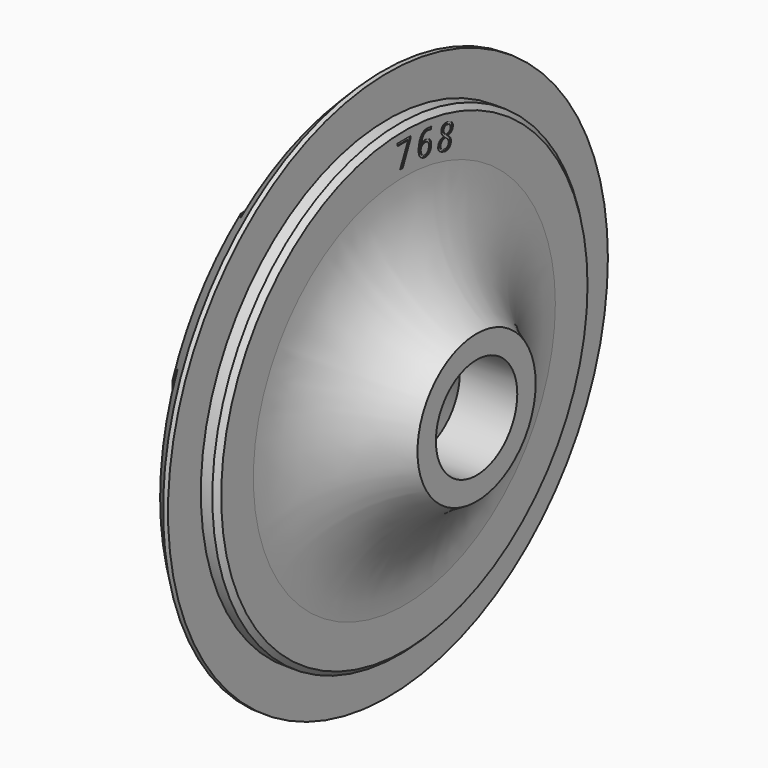
from build123d import *

# Parameters (mm, degrees)
F2_SIZE      = 1.3
F4_DEPTH     = 0.4
F5_T1_DEPTH  = 0.4
F5_T3_DEPTH  = 1.1640297733
F6_TEXT_SIZE = 2.0833333333
F7_DEPTH     = 0.05
F8_SIZE      = 0.3
F9_SIZE      = 0.1


# Not quite as in the source:
# - a fillet or chamfer that OpenCascade refuses, or shapes differently, is made with other operations: its cross-section is extruded or revolved along the edge and cut away or added
# - Text() gives the source's letters only with a copy of the font that has no kerning and outlines rounded to 1/6400 em; it was checked with that copy


with BuildPart() as f1:
    # F0 (on Top) → F1 (revolve)
    with BuildSketch(Plane.XY):
        with BuildLine():
            Line((-4.4, 11.5), (-4.4, 14.25))
            Line((-4.4, 14.25), (-5.4, 14.25))
            Line((-5.4, 14.25), (-5.4, 16.75))
            Line((-5.4, 16.75), (-7, 16.75))
            Line((-7, 16.75), (-7, 6))
            Line((-7, 6), (-6.4, 6))
            Line((-6.4, 6), (-3.5, 3.1))
            Line((-3.5, 3.1), (0, 3.1))
            Line((0, 3.1), (0, 4.5))
            ThreePointArc((0, 4.5), (-3.20864483, 7.3659946783), (-4.4, 11.5))
        make_face()
    revolve(axis=Axis((-3.5, 0, 0), (-1, 0, 0)))

    # F2
    f2_edges = [f1.edges().sort_by_distance(p)[0] for p in [
        (-7, -16.75, 0),
    ]]
    chamfer(f2_edges, length=F2_SIZE)

    # F3 (on face) → F4 (cut)
    with BuildSketch(Plane(origin=(-7, 0, 0), x_dir=(0, -1, 0), z_dir=(-1, 0, 0))):
        with BuildLine():
            ThreePointArc((14.5, -8.3852549156), (16.1777238819, -4.3409388385), (16.75, 0))
            ThreePointArc((16.75, 0), (16.1777238819, 4.3409388385), (14.5, 8.3852549156))
            Line((14.5, 8.3852549156), (14.5, 5.3340884882))
            ThreePointArc((14.5, 5.3340884882), (15.2106459429, 2.7090127353), (15.45, 0))
            ThreePointArc((15.45, 0), (15.2106459429, -2.7090127353), (14.5, -5.3340884882))
            Line((14.5, -5.3340884882), (14.5, -8.3852549156))
        make_face()
        with BuildLine():
            Line((9.0803358969, 12.5), (11.1495515605, 12.5))
            ThreePointArc((11.1495515605, 12.5), (0, 16.75), (-11.1495515605, 12.5))
            Line((-11.1495515605, 12.5), (-9.0803358969, 12.5))
            ThreePointArc((-9.0803358969, 12.5), (0, 15.45), (9.0803358969, 12.5))
        make_face()
        with BuildLine():
            ThreePointArc((15.45, 0), (15.2106459429, 2.7090127353), (14.5, 5.3340884882))
            Line((14.5, 5.3340884882), (14.5, -5.3340884882))
            ThreePointArc((14.5, -5.3340884882), (15.2106459429, -2.7090127353), (15.45, 0))
        make_face()
        with BuildLine():
            ThreePointArc((2.9, -16.49704519), (5.9018735713, -15.6757898796), (8.7, -14.3133678776))
            Line((8.7, -14.3133678776), (8.7, -12.7676348632))
            ThreePointArc((8.7, -12.7676348632), (5.9236241205, -14.2693089279), (2.9, -15.1753912635))
            Line((2.9, -15.1753912635), (2.9, -16.49704519))
        make_face()
        with BuildLine():
            Line((8.7, 12.5), (9.0803358969, 12.5))
            ThreePointArc((9.0803358969, 12.5), (0, 15.45), (-9.0803358969, 12.5))
            Line((-9.0803358969, 12.5), (-8.7, 12.5))
            Line((-8.7, 12.5), (-4.9428840308, 6.2471089796))
            ThreePointArc((-4.9428840308, 6.2471089796), (-3.7060377863, 5.7536573635), (-2.9, 6.813650862))
            Line((-2.9, 6.813650862), (-2.9, 12.5))
            Line((-2.9, 12.5), (2.9, 12.5))
            Line((2.9, 12.5), (2.9, 6.813650862))
            ThreePointArc((2.9, 6.813650862), (3.7060377863, 5.7536573635), (4.9428840308, 6.2471089796))
            Line((4.9428840308, 6.2471089796), (8.7, 12.5))
        make_face()
        with BuildLine():
            ThreePointArc((2.9, -15.1753912635), (5.9236241205, -14.2693089279), (8.7, -12.7676348632))
            Line((8.7, -12.7676348632), (8.7, 1.2386966468))
            Line((8.7, 1.2386966468), (2.9, -8.4141243508))
            Line((2.9, -8.4141243508), (2.9, -15.1753912635))
        make_face()
        with BuildLine():
            Line((-14.5, 5.3340884882), (-14.5, 8.3852549156))
            ThreePointArc((-14.5, 8.3852549156), (-16.75, 0), (-14.5, -8.3852549156))
            Line((-14.5, -8.3852549156), (-14.5, -5.3340884882))
            ThreePointArc((-14.5, -5.3340884882), (-15.45, 0), (-14.5, 5.3340884882))
        make_face()
        with BuildLine():
            ThreePointArc((-8.7, -14.3133678776), (-5.9018735713, -15.6757898796), (-2.9, -16.49704519))
            Line((-2.9, -16.49704519), (-2.9, -15.1753912635))
            ThreePointArc((-2.9, -15.1753912635), (-5.9236241205, -14.2693089279), (-8.7, -12.7676348632))
            Line((-8.7, -12.7676348632), (-8.7, -14.3133678776))
        make_face()
        with BuildLine():
            Line((-14.5, -5.3340884882), (-14.5, 5.3340884882))
            ThreePointArc((-14.5, 5.3340884882), (-15.45, 0), (-14.5, -5.3340884882))
        make_face()
        with BuildLine():
            ThreePointArc((-8.7, -12.7676348632), (-5.9236241205, -14.2693089279), (-2.9, -15.1753912635))
            Line((-2.9, -15.1753912635), (-2.9, -8.4141243508))
            Line((-2.9, -8.4141243508), (-8.7, 1.2386966468))
            Line((-8.7, 1.2386966468), (-8.7, -12.7676348632))
        make_face()
    extrude(amount=-F4_DEPTH, mode=Mode.SUBTRACT)

    # F5: fillet of radius 1.1 on 4 edges, made by hand

    # F5_s2 → F5_t1 (join)
    with BuildSketch(Plane.YZ.offset(-7)):
        with BuildLine():
            ThreePointArc((8.7004, -2.7283019394), (7.8939620715, -1.6677822271), (6.6565018181, -2.161478808))
            Line((6.6565018181, -2.161478808), (6.5621666073, -2.1047964949))
            ThreePointArc((6.5621666073, -2.1047964949), (7.5840871317, -0.4048117751), (8.6056647892, 1.29537896))
            Line((8.6056647892, 1.29537896), (8.8100546074, 1.2386966468))
            ThreePointArc((8.8100546074, 1.2386966468), (8.8100546074, -0.7448026463), (8.8104546074, -2.7283019394))
            Line((8.8104546074, -2.7283019394), (8.7004, -2.7283019394))
        make_face()
        with BuildLine():
            ThreePointArc((-8.7004, -2.7283019394), (-7.8939620715, -1.6677822271), (-6.6565018181, -2.161478808))
            Line((-6.6565018181, -2.161478808), (-6.5621666073, -2.1047964949))
            ThreePointArc((-6.5621666073, -2.1047964949), (-7.5840871317, -0.4048117751), (-8.6056647892, 1.29537896))
            Line((-8.6056647892, 1.29537896), (-8.8100546074, 1.2386966468))
            ThreePointArc((-8.8100546074, 1.2386966468), (-8.8100546074, -0.7448026463), (-8.8104546074, -2.7283019394))
            Line((-8.8104546074, -2.7283019394), (-8.7004, -2.7283019394))
        make_face()
    extrude(amount=F5_T1_DEPTH)

    # F5_s4 → F5_t3 (join)
    with BuildSketch(Plane.YZ.offset(-7)):
        with BuildLine():
            ThreePointArc((2.8996, -8.7197359984), (2.9396937884, -8.4251324126), (3.0570587677, -8.1519580246))
            Line((3.0570587677, -8.1519580246), (2.9625646445, -8.0951802272))
            ThreePointArc((2.9625646445, -8.0951802272), (2.8842066941, -8.2263663979), (2.8055058768, -8.3573465534))
            Line((2.8055058768, -8.3573465534), (2.78976, -8.4141243508))
            ThreePointArc((2.78976, -8.4141243508), (2.78976, -8.5669301746), (2.78936, -8.7197359984))
            Line((2.78936, -8.7197359984), (2.8996, -8.7197359984))
        make_face()
        with BuildLine():
            ThreePointArc((-2.8996, -8.7197359984), (-2.9396937884, -8.4251324126), (-3.0570587677, -8.1519580246))
            Line((-3.0570587677, -8.1519580246), (-2.9625646445, -8.0951802272))
            ThreePointArc((-2.9625646445, -8.0951802272), (-2.8842066941, -8.2263663979), (-2.8055058768, -8.3573465534))
            Line((-2.8055058768, -8.3573465534), (-2.78976, -8.4141243508))
            ThreePointArc((-2.78976, -8.4141243508), (-2.78976, -8.5669301746), (-2.78936, -8.7197359984))
            Line((-2.78936, -8.7197359984), (-2.8996, -8.7197359984))
        make_face()
    extrude(amount=F5_T3_DEPTH)

    # F6 (on face) → F7 (cut)
    with BuildSketch(Plane.YZ.offset(-4.4)):
        with Locations((-0.6101888021, 12)):
            Text('7', F6_TEXT_SIZE, font='Open Sans', text_align=(TextAlign.LEFT, TextAlign.BOTTOM))
        with BuildLine():
            add(Edge.make_bspline(
                [(1.3911920227, 11.9124736168), (1.2492672408, 11.965505738), (1.168086207, 12.102022835)],
                knots=[0.2780169607, 0.2780169607, 0.2780169607, 1, 1, 1], degree=2))
            Line((1.3911920227, 11.9124736168), (1.5039988028, 11.9053764158))
            Line((1.5039988028, 11.9053764158), (1.6329910314, 11.8807698321))
            add(Edge.make_bspline(
                [(1.8658957751, 11.9728554781), (1.7668517571, 11.8921760098), (1.6329910314, 11.8807698321)],
                knots=[0, 0, 0, 0.6961452699, 0.6961452699, 0.6961452699], degree=2))
            add(Edge.make_bspline(
                [(2.0372600894, 12.3190162698), (2.0081707028, 12.0887500648), (1.8658957751, 11.9728554781)],
                knots=[0, 0, 0, 1, 1, 1], degree=2))
            add(Edge.make_bspline(
                [(1.9639386607, 12.6593399563), (2.063248784, 12.5247379706), (2.0372600894, 12.3190162698)],
                knots=[0, 0, 0, 1, 1, 1], degree=2))
            add(Edge.make_bspline(
                [(1.6656888708, 12.8190738665), (1.8646285374, 12.7939419421), (1.9639386607, 12.6593399563)],
                knots=[0, 0, 0, 1, 1, 1], degree=2))
            add(Edge.make_bspline(
                [(1.2923652787, 12.6897134657), (1.4254110915, 12.849428009), (1.6656888708, 12.8190738665)],
                knots=[0, 0, 0, 1, 1, 1], degree=2))
            Line((1.2923652787, 12.6897134657), (1.2804159806, 12.6912230132))
            add(Edge.make_bspline(
                [(1.4762395094, 13.1387963058), (1.332429483, 13.006854298), (1.2804159806, 12.6912230132)],
                knots=[0, 0, 0, 1, 1, 1], degree=2))
            add(Edge.make_bspline(
                [(1.8574207289, 13.2407513582), (1.6200495358, 13.2707383135), (1.4762395094, 13.1387963058)],
                knots=[0, 0, 0, 1, 1, 1], degree=2))
            add(Edge.make_bspline(
                [(2.0318631422, 13.1931217276), (1.9572135163, 13.2281445974), (1.8574207289, 13.2407513582)],
                knots=[0, 0, 0, 1, 1, 1], degree=2))
            Line((2.0318631422, 13.1931217276), (2.0501001068, 13.3374821676))
            add(Edge.make_bspline(
                [(1.8729447966, 13.3792204636), (1.9869475601, 13.3648185653), (2.0501001068, 13.3374821676)],
                knots=[0, 0, 0, 1, 1, 1], degree=2))
            add(Edge.make_bspline(
                [(1.3456378689, 13.2269867417), (1.5419169421, 13.4210390067), (1.8729447966, 13.3792204636)],
                knots=[0, 0, 0, 1, 1, 1], degree=2))
            add(Edge.make_bspline(
                [(1.0944031103, 12.5979154329), (1.1493587957, 13.0329344767), (1.3456378689, 13.2269867417)],
                knots=[0, 0, 0, 1, 1, 1], degree=2))
            add(Edge.make_bspline(
                [(1.168086207, 12.102022835), (1.0556444606, 12.2911091288), (1.0944031103, 12.5979154329)],
                knots=[0, 0, 0, 1, 1, 1], degree=2))
        make_face()
        with BuildLine():
            add(Edge.make_bspline(
                [(1.5255567916, 12.0266778564), (1.6689483695, 12.0085632875), (1.7594957026, 12.088994757)],
                knots=[0, 0, 0, 1, 1, 1], degree=2))
            add(Edge.make_bspline(
                [(1.3631201393, 12.100515938), (1.4306083143, 12.0386726385), (1.5255567916, 12.0266778564)],
                knots=[0, 0, 0, 1, 1, 1], degree=2))
            add(Edge.make_bspline(
                [(1.2666047187, 12.2572402731), (1.2956319644, 12.1623592375), (1.3631201393, 12.100515938)],
                knots=[0, 0, 0, 1, 1, 1], degree=2))
            add(Edge.make_bspline(
                [(1.2507146153, 12.456112498), (1.237577473, 12.3521213086), (1.2666047187, 12.2572402731)],
                knots=[0, 0, 0, 1, 1, 1], degree=2))
            add(Edge.make_bspline(
                [(1.3128222221, 12.5867280854), (1.259649504, 12.526839425), (1.2507146153, 12.456112498)],
                knots=[0, 0, 0, 1, 1, 1], degree=2))
            add(Edge.make_bspline(
                [(1.4464602893, 12.6745121437), (1.3659949402, 12.6466167459), (1.3128222221, 12.5867280854)],
                knots=[0, 0, 0, 1, 1, 1], degree=2))
            add(Edge.make_bspline(
                [(1.6176757137, 12.6909431409), (1.5269256385, 12.7024075415), (1.4464602893, 12.6745121437)],
                knots=[0, 0, 0, 1, 1, 1], degree=2))
            add(Edge.make_bspline(
                [(1.8270201595, 12.5793527447), (1.7639738776, 12.6724613848), (1.6176757137, 12.6909431409)],
                knots=[0, 0, 0, 1, 1, 1], degree=2))
            add(Edge.make_bspline(
                [(1.8715846852, 12.3399459407), (1.8900664413, 12.4862441047), (1.8270201595, 12.5793527447)],
                knots=[0, 0, 0, 1, 1, 1], degree=2))
            add(Edge.make_bspline(
                [(1.7594957026, 12.088994757), (1.8500430357, 12.1694262264), (1.8715846852, 12.3399459407)],
                knots=[0, 0, 0, 1, 1, 1], degree=2))
        make_face(mode=Mode.SUBTRACT)
        with BuildLine():
            Line((2.984278646, 11.6229979335), (3.1084826292, 11.582641613))
            add(Edge.make_bspline(
                [(3.3407163455, 11.6244062371), (3.239004536, 11.5744991717), (3.1084826292, 11.582641613)],
                knots=[0, 0, 0, 0.666283244, 0.666283244, 0.666283244], degree=2))
            add(Edge.make_bspline(
                [(3.5393535811, 11.8783969056), (3.4933718571, 11.6993099149), (3.3407163455, 11.6244062371)],
                knots=[0, 0, 0, 1, 1, 1], degree=2))
            add(Edge.make_bspline(
                [(3.5202228201, 12.1108345939), (3.5705207707, 11.9997850947), (3.5393535811, 11.8783969056)],
                knots=[0, 0, 0, 1, 1, 1], degree=2))
            add(Edge.make_bspline(
                [(3.3161551014, 12.3507625756), (3.4699248695, 12.2218840932), (3.5202228201, 12.1108345939)],
                knots=[0, 0, 0, 1, 1, 1], degree=2))
            add(Edge.make_bspline(
                [(3.568049378, 12.4561432869), (3.4796477929, 12.385410887), (3.3161551014, 12.3507625756)],
                knots=[0, 0, 0, 1, 1, 1], degree=2))
            add(Edge.make_bspline(
                [(3.683813327, 12.633445058), (3.6564509631, 12.5268756868), (3.568049378, 12.4561432869)],
                knots=[0, 0, 0, 1, 1, 1], degree=2))
            add(Edge.make_bspline(
                [(3.6335387466, 12.9160570829), (3.7252616415, 12.7948755848), (3.683813327, 12.633445058)],
                knots=[0, 0, 0, 1, 1, 1], degree=2))
            add(Edge.make_bspline(
                [(3.3447571031, 13.0878346681), (3.5418158517, 13.037238581), (3.6335387466, 12.9160570829)],
                knots=[0, 0, 0, 1, 1, 1], degree=2))
            add(Edge.make_bspline(
                [(3.0109417502, 13.0744004645), (3.1505360004, 13.1377021715), (3.3447571031, 13.0878346681)],
                knots=[0, 0, 0, 1, 1, 1], degree=2))
            add(Edge.make_bspline(
                [(2.8311134914, 12.8543976406), (2.8713474999, 13.0110987574), (3.0109417502, 13.0744004645)],
                knots=[0, 0, 0, 1, 1, 1], degree=2))
            add(Edge.make_bspline(
                [(2.838987399, 12.6396377139), (2.8027796827, 12.7440447413), (2.8311134914, 12.8543976406)],
                knots=[0, 0, 0, 1, 1, 1], degree=2))
            add(Edge.make_bspline(
                [(2.9914150698, 12.4237231833), (2.8751951154, 12.5352306864), (2.838987399, 12.6396377139)],
                knots=[0, 0, 0, 1, 1, 1], degree=2))
            add(Edge.make_bspline(
                [(2.5910685385, 12.1158256928), (2.6545362701, 12.363016187), (2.9914150698, 12.4237231833)],
                knots=[0, 0, 0, 1, 1, 1], degree=2))
            add(Edge.make_bspline(
                [(2.6417479014, 11.7974853225), (2.5434677398, 11.9304328221), (2.5910685385, 12.1158256928)],
                knots=[0, 0, 0, 1, 1, 1], degree=2))
            add(Edge.make_bspline(
                [(2.8349707002, 11.6514799475), (2.7081685053, 11.7076355191), (2.6417479014, 11.7974853225)],
                knots=[0.3241707912, 0.3241707912, 0.3241707912, 1, 1, 1], degree=2))
            Line((2.8349707002, 11.6514799475), (2.984278646, 11.6229979335))
        make_face()
        with BuildLine():
            add(Edge.make_bspline(
                [(2.7517619607, 12.0701976025), (2.7214043085, 11.9519623534), (2.7865785865, 11.8648198118)],
                knots=[0, 0, 0, 1, 1, 1], degree=2))
            add(Edge.make_bspline(
                [(2.864611575, 12.2361487897), (2.7791243246, 12.1767669738), (2.7517619607, 12.0701976025)],
                knots=[0, 0, 0, 1, 1, 1], degree=2))
            add(Edge.make_bspline(
                [(3.1132165763, 12.3208649627), (2.9500988255, 12.2955306057), (2.864611575, 12.2361487897)],
                knots=[0, 0, 0, 1, 1, 1], degree=2))
            add(Edge.make_bspline(
                [(3.3441396618, 12.1076496333), (3.2863130088, 12.2018117292), (3.1132165763, 12.3208649627)],
                knots=[0, 0, 0, 1, 1, 1], degree=2))
            add(Edge.make_bspline(
                [(3.3774373318, 11.9179534561), (3.4019663148, 12.0134875375), (3.3441396618, 12.1076496333)],
                knots=[0, 0, 0, 1, 1, 1], degree=2))
            add(Edge.make_bspline(
                [(3.2470462958, 11.7497845528), (3.3465939571, 11.797826443), (3.3774373318, 11.9179534561)],
                knots=[0, 0, 0, 1, 1, 1], degree=2))
            add(Edge.make_bspline(
                [(3.0005716315, 11.7394671052), (3.1474986344, 11.7017426627), (3.2470462958, 11.7497845528)],
                knots=[0, 0, 0, 1, 1, 1], degree=2))
            add(Edge.make_bspline(
                [(2.7865785865, 11.8648198118), (2.8517528645, 11.7776772701), (3.0005716315, 11.7394671052)],
                knots=[0, 0, 0, 1, 1, 1], degree=2))
        make_face(mode=Mode.SUBTRACT)
        with BuildLine():
            add(Edge.make_bspline(
                [(3.3087838148, 12.9555816174), (3.1855038617, 12.9872345295), (3.1003297681, 12.9460886351)],
                knots=[0, 0, 0, 1, 1, 1], degree=2))
            add(Edge.make_bspline(
                [(3.4903122269, 12.8464622774), (3.4339555319, 12.9234429829), (3.3087838148, 12.9555816174)],
                knots=[0, 0, 0, 1, 1, 1], degree=2))
            add(Edge.make_bspline(
                [(3.5210875403, 12.6698486686), (3.5466689219, 12.7694815719), (3.4903122269, 12.8464622774)],
                knots=[0, 0, 0, 1, 1, 1], degree=2))
            add(Edge.make_bspline(
                [(3.4217231258, 12.5263131832), (3.4978538171, 12.5793592912), (3.5210875403, 12.6698486686)],
                knots=[0, 0, 0, 1, 1, 1], degree=2))
            add(Edge.make_bspline(
                [(3.1895176683, 12.4504934191), (3.3455924345, 12.4732670752), (3.4217231258, 12.5263131832)],
                knots=[0, 0, 0, 1, 1, 1], degree=2))
            add(Edge.make_bspline(
                [(3.0080382263, 12.6357221665), (3.0494930217, 12.5556779911), (3.1895176683, 12.4504934191)],
                knots=[0, 0, 0, 1, 1, 1], degree=2))
            add(Edge.make_bspline(
                [(2.989817154, 12.8062557193), (2.9665834309, 12.7157663419), (3.0080382263, 12.6357221665)],
                knots=[0, 0, 0, 1, 1, 1], degree=2))
            add(Edge.make_bspline(
                [(3.1003297681, 12.9460886351), (3.0151556744, 12.9049427406), (2.989817154, 12.8062557193)],
                knots=[0, 0, 0, 1, 1, 1], degree=2))
        make_face(mode=Mode.SUBTRACT)
    extrude(amount=-F7_DEPTH, mode=Mode.SUBTRACT)

    # F8
    f8_edges = [f1.edges().sort_by_distance(p)[0] for p in [
        (-4.4, -14.25, 0),
    ]]
    chamfer(f8_edges, length=F8_SIZE)

    # F9
    f9_edges = [f1.edges().sort_by_distance(p)[0] for p in [
        (-7, 8.7, -7.733134),
        (-7, 7.893962, -1.667782),
        (-7, -2.9, -11.932716),
        (-7, -2.939694, -8.425132),
        (-7, -4.857117, -5.156935),
        (-7, -7.893962, -1.667782),
        (-7, -14.5, 0),
        (-7, 6.821442, 9.373554),
        (-7, 3.706038, 5.753657),
        (-7, 2.9, 9.656825),
        (-7, -2.9, 9.656825),
        (-7, -3.706038, 5.753657),
        (-7, -6.821442, 9.373554),
        (-7, 4.857117, -5.156935),
        (-7, 2.939694, -8.425132),
        (-7, 2.9, -11.932716),
        (-7, -8.7, -7.733134),
        (-7, 0, 12.5),
        (-7, 8.890168, 12.5),
        (-7, -8.890168, 12.5),
        (-7, 14.5, 0),
    ]]
    chamfer(f9_edges, length=F9_SIZE)


solid = f1.part
